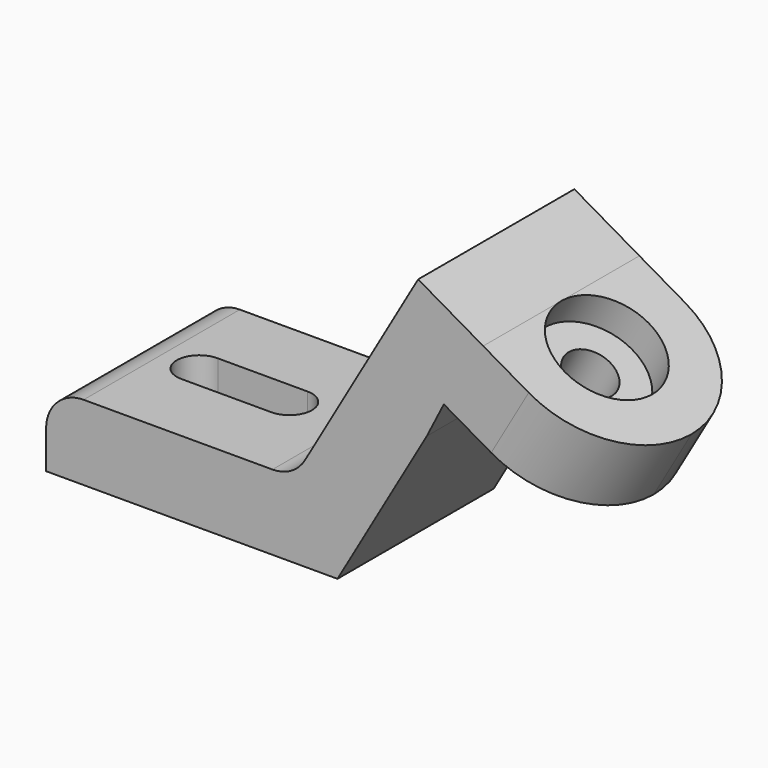
from build123d import *

# Parameters (mm, degrees)
F1_DEPTH = 26
F3_DEPTH = 10.001
F4_R     = 12.99999
F5_R     = 7
F6_DEPTH = 4.4
F7_R     = 3.3
F8_DEPTH = 53.801


# Not quite as in the source:
# - a fillet or chamfer is up to 0.001 mm smaller than in the source, because OpenCascade refuses the exact size


with BuildPart() as f1:
    # F0 (on Front) → F1 (new body)
    with BuildSketch(Plane.XZ):
        with BuildLine():
            Line((-38.8, 0), (0, 0))
            Line((0, 0), (11.9, 20.6114046101))
            Line((11.9, 20.6114046101), (14.1603821252, 25.0713006457))
            Line((14.1603821252, 25.0713006457), (18.7301270189, 22.441531629))
            Line((18.7301270189, 22.441531629), (31.7205080757, 14.941531629))
            Line((31.7205080757, 14.941531629), (36.7205080757, 23.6017856668))
            Line((36.7205080757, 23.6017856668), (19.4, 33.6017856668))
            Line((19.4, 33.6017856668), (10.7397459622, 38.6017856668))
            Line((10.7397459622, 38.6017856668), (-4.3301270189, 12.5))
            ThreePointArc((-4.3301270189, 12.5), (-6.1602540378, 10.6698729811), (-8.6602540378, 10))
            Line((-8.6602540378, 10), (-33.8, 10))
            ThreePointArc((-33.8, 10), (-37.3355339059, 8.5355339059), (-38.8, 5))
            Line((-38.8, 5), (-38.8, 0))
        make_face()
    extrude(amount=F1_DEPTH)

    # F2 (on face) → F3 (cut, through all)
    with BuildSketch(Plane.XY.offset(10)):
        with BuildLine():
            ThreePointArc((-28.7603622502, -15.99973813), (-26.6647115828, -15.1072596839), (-25.8, -13))
            ThreePointArc((-25.8, -13), (-26.6495430639, -10.9082220563), (-28.7170233106, -10.0011477414))
            ThreePointArc((-28.7170233106, -10.0011477414), (-31.7993750812, -12.9387699222), (-28.839480247, -15.9997402071))
            Line((-28.839480247, -15.9997402071), (-28.7603622502, -15.99973813))
        make_face()
        with BuildLine():
            ThreePointArc((-28.7170233106, -10.0011477414), (-26.6495430639, -10.9082220563), (-25.8, -13))
            ThreePointArc((-25.8, -13), (-26.6647115828, -15.1072596839), (-28.7603622502, -15.99973813))
            Line((-28.7603622502, -15.99973813), (-16.7999212569, -15.9994241356))
            ThreePointArc((-16.7999212569, -15.9994241356), (-19.7994241345, -13.0001113407), (-16.8001439382, -10.0005758668))
            Line((-16.8001439382, -10.0005758668), (-28.7170233106, -10.0011477414))
        make_face()
        with BuildLine():
            ThreePointArc((-28.839480247, -15.9997402071), (-28.7999212418, -15.999999999), (-28.7603622502, -15.99973813))
            Line((-28.7603622502, -15.99973813), (-28.839480247, -15.9997402071))
        make_face()
        with BuildLine():
            ThreePointArc((-13.8005758634, -13), (-14.6791377438, -10.8790359641), (-16.8001439382, -10.0005758668))
            ThreePointArc((-16.8001439382, -10.0005758668), (-19.7994241345, -13.0001113407), (-16.7999212569, -15.9994241356))
            ThreePointArc((-16.7999212569, -15.9994241356), (-14.6790590136, -15.1208853066), (-13.8005758634, -13))
        make_face()
    extrude(amount=-F3_DEPTH, mode=Mode.SUBTRACT)

    # F4 (radius 13 in the source; OpenCascade refuses exactly that, so slightly less here)
    f4_edges = [f1.edges().sort_by_distance(p)[0] for p in [
        (34.220508, -26, 19.271659),
        (34.220508, 0, 19.271659),
    ]]
    fillet(f4_edges, radius=F4_R)

    # F5 (on face) → F6 (cut)
    with BuildSketch(Plane(origin=(19.4, 0, 33.6017856668), x_dir=(0.8660254038, 0, -0.5), z_dir=(0.5, 0, 0.8660254038))):
        with Locations((7, -13)):
            Circle(F5_R)
    extrude(amount=-F6_DEPTH, mode=Mode.SUBTRACT)

    # F7 (on face) → F8 (cut, through all)
    with BuildSketch(Plane(origin=(17.2, 0, 29.7912738902), x_dir=(0.8660254038, 0, -0.5), z_dir=(0.5, 0, 0.8660254038))):
        with Locations((7, -13)):
            Circle(F7_R)
    extrude(amount=-F8_DEPTH, mode=Mode.SUBTRACT)


solid = f1.part
